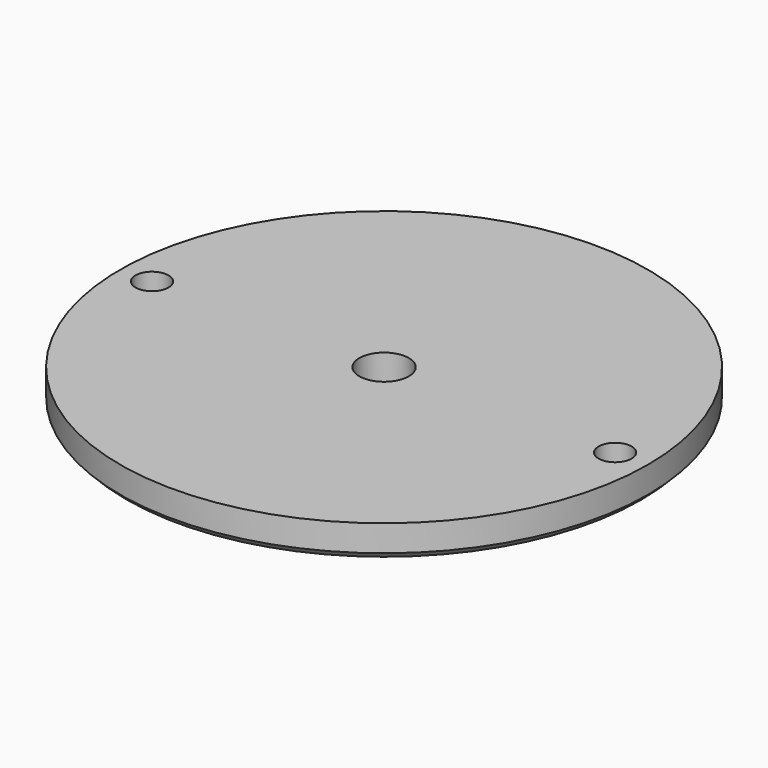
from build123d import *

# Parameters (mm, degrees)
F0_R     = 50.8
F1_DEPTH = 6.35
F2_R     = 4.7625
F2_R_2   = 3.175
F3_DEPTH = 25.4
F4_SIZE  = 1.27


# Not quite as in the source:
# - a length typed as a fraction of an inch, garbled in the dataset ("3 / 203.2 mm" for 3/8 in), is restored


with BuildPart() as f1:
    # F0 (on Top) → F1 (new body)
    with BuildSketch(Plane.XY):
        Circle(F0_R)
    extrude(amount=F1_DEPTH)

    # F2 (on Top) → F3 (cut)
    with BuildSketch(Plane.XY):
        Circle(F2_R)
        with Locations((-44.6634478867, 0)):
            Circle(F2_R_2)
        with Locations((44.4713458419, 0)):
            Circle(F2_R_2)
    extrude(amount=F3_DEPTH, mode=Mode.SUBTRACT)

    # F4
    f4_edges = [f1.edges().sort_by_distance(p)[0] for p in [
        (-50.8, 0, 0),
    ]]
    chamfer(f4_edges, length=F4_SIZE)


solid = f1.part
